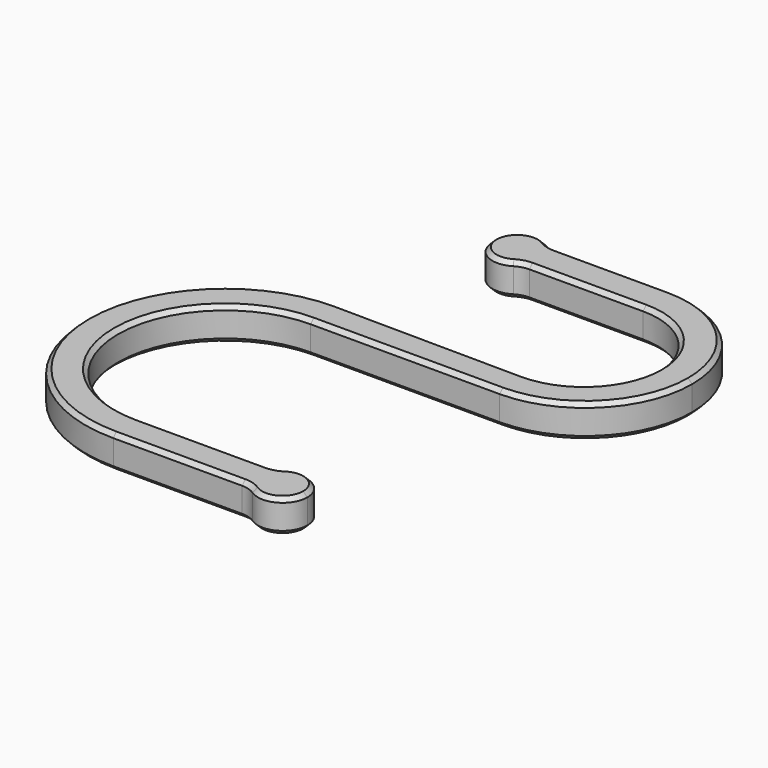
from build123d import *

# Parameters (mm, degrees)
F1_DEPTH = 4
F2_R     = 3
F3_SIZE  = 0.5


with BuildPart() as f1:
    # F0 (on Top) → F1 (new body)
    with BuildSketch(Plane.XY):
        with BuildLine():
            Line((0.2956298201, 16.9974293059), (0, 17))
            ThreePointArc((0, 17), (-17, 0), (0, -17))
            ThreePointArc((0, -17), (5.8309518948, -15.9687194227), (10.9544511501, -13))
            Line((10.9544511501, -13), (0, -13))
            ThreePointArc((0, -13), (-13, 0), (0, 13))
            Line((0, 13), (10.9544511501, 13))
            ThreePointArc((10.9544511501, 13), (5.9695846357, 15.9174137119), (0.2956298201, 16.9974293059))
        make_face()
        with BuildLine():
            ThreePointArc((10.9544511501, -13), (5.8309518948, -15.9687194227), (0, -17))
            Line((0, -17), (16.7639320225, -17))
            ThreePointArc((16.7639320225, -17), (16, -15), (16.7639320225, -13))
            Line((16.7639320225, -13), (10.9544511501, -13))
        make_face()
        with BuildLine():
            Line((13.73523492, 16.8805631746), (0.2956298201, 16.9974293059))
            ThreePointArc((0.2956298201, 16.9974293059), (5.9695846357, 15.9174137119), (10.9544511501, 13))
            Line((10.9544511501, 13), (23, 13))
            ThreePointArc((23, 13), (17.9776837381, 14.0093228146), (13.73523492, 16.8805631746))
        make_face()
        with BuildLine():
            ThreePointArc((16.7639320225, -13), (16, -15), (16.7639320225, -17))
            Line((16.7639320225, -17), (19, -17))
            Line((19, -17), (19, -13))
            Line((19, -13), (16.7639320225, -13))
        make_face()
        with BuildLine():
            Line((19, -17), (16.7639320225, -17))
            ThreePointArc((16.7639320225, -17), (20.0704662693, -17.8025170769), (22, -15))
            ThreePointArc((22, -15), (20.0704662693, -12.1974829231), (16.7639320225, -13))
            Line((16.7639320225, -13), (19, -13))
            Line((19, -13), (19, -17))
        make_face()
        with BuildLine():
            Line((22.8434900953, 16.8013609557), (13.73523492, 16.8805631746))
            ThreePointArc((13.73523492, 16.8805631746), (17.9776837381, 14.0093228146), (23, 13))
            ThreePointArc((23, 13), (32.1923881554, 16.8076118446), (36, 26))
            ThreePointArc((36, 26), (32.1923881554, 35.1923881554), (23, 39))
            ThreePointArc((23, 39), (17.775059809, 37.903780912), (13.4313010289, 34.8))
            Line((13.4313010289, 34.8), (23, 34.8))
            ThreePointArc((23, 34.8), (29.3639610307, 32.1639610307), (32, 25.8))
            ThreePointArc((32, 25.8), (29.3639610307, 19.4360389693), (23, 16.8))
            ThreePointArc((23, 16.8), (22.9217420891, 16.8003402454), (22.8434900953, 16.8013609557))
        make_face()
        with BuildLine():
            Line((8.1424285286, 34.8), (13.4313010289, 34.8))
            ThreePointArc((13.4313010289, 34.8), (17.775059809, 37.903780912), (23, 39))
            Line((23, 39), (8.1424285286, 39))
            ThreePointArc((8.1424285286, 39), (8.7773445578, 38.0341768853), (9, 36.9))
            ThreePointArc((9, 36.9), (8.7773445578, 35.7658231147), (8.1424285286, 34.8))
        make_face()
        with BuildLine():
            ThreePointArc((8.1424285286, 39), (3, 36.9), (8.1424285286, 34.8))
            Line((8.1424285286, 34.8), (6, 34.8))
            Line((6, 34.8), (6, 39))
            Line((6, 39), (8.1424285286, 39))
        make_face()
        with BuildLine():
            Line((6, 34.8), (8.1424285286, 34.8))
            ThreePointArc((8.1424285286, 34.8), (8.7773445578, 35.7658231147), (9, 36.9))
            ThreePointArc((9, 36.9), (8.7773445578, 38.0341768853), (8.1424285286, 39))
            Line((8.1424285286, 39), (6, 39))
            Line((6, 39), (6, 34.8))
        make_face()
    extrude(amount=F1_DEPTH)

    # F2
    f2_edges = [f1.edges().sort_by_distance(p)[0] for p in [
        (16.763932, -17, 2),
        (8.142429, 34.8, 2),
        (16.763932, -13, 2),
        (8.142429, 39, 2),
    ]]
    fillet(f2_edges, radius=F2_R)

    # F3
    f3_edges = [f1.edges().sort_by_distance(p)[0] for p in [
        (7.841688, -17, 4),
        (7.841688, -13, 4),
        (-13, 0, 4),
        (-17, 0, 4),
        (11.5, 13, 4),
        (11.421745, 16.90068, 4),
        (22, -15, 4),
        (16.549401, -12.872281, 4),
        (16.549401, -17.127719, 4),
        (36, 26, 4),
        (31.99966, 25.721742, 4),
        (16.080348, 34.8, 4),
        (16.080348, 39, 4),
        (8.339112, 34.685308, 4),
        (8.339112, 39.114692, 4),
        (3, 36.9, 4),
        (22, -15, 0),
        (16.549401, -17.127719, 0),
        (7.841688, -13, 0),
        (7.841688, -17, 0),
        (16.549401, -12.872281, 0),
        (-13, 0, 0),
        (-17, 0, 0),
        (11.5, 13, 0),
        (11.421745, 16.90068, 0),
        (31.99966, 25.721742, 0),
        (16.080348, 34.8, 0),
        (8.339112, 34.685308, 0),
        (3, 36.9, 0),
        (36, 26, 0),
        (8.339112, 39.114692, 0),
        (16.080348, 39, 0),
    ]]
    chamfer(f3_edges, length=F3_SIZE)


solid = f1.part
